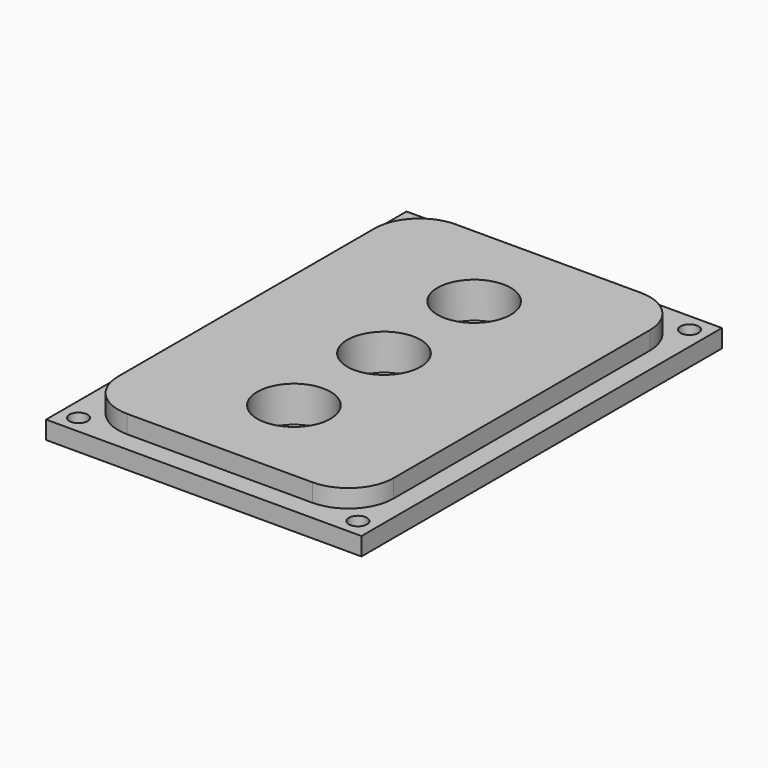
from build123d import *

# Parameters (mm, degrees)
F0_W            = 70
F0_H            = 100
F2_DEPTH        = 4
F1_W            = 61.1
F1_H            = 91.1
F3_DEPTH        = 4
F5_D            = 16.25
F5_DEPTH        = 10
F5_TIP          = 4.8819925296
F6_TEXT_SIZE    = 9.5338899996
F7_DEPTH        = 0.5
F9_R            = 10
F10_D           = 4
F10_DEPTH       = 10
F10_CSINK_D     = 5
F10_CSINK_ANGLE = 90
F10_TIP         = 1.2017212381


# Not quite as in the source:
# - Text() gives the source's letters only with a copy of the font that has no kerning and outlines rounded to 1/6400 em; it was checked with that copy


with BuildPart() as f2:
    # F0 (on Top) → F2 (new body)
    with BuildSketch(Plane.XY):
        Rectangle(F0_W, F0_H)
    extrude(amount=-F2_DEPTH)

    # F1 (on Top) → F3 (join)
    with BuildSketch(Plane.XY):
        Rectangle(F1_W, F1_H)
    extrude(amount=F3_DEPTH)

    # F5
    with Locations(Plane(origin=(0, 0, -4), x_dir=(1, 0, 0), z_dir=(0, 0, -1))):
        with Locations((0, 25), (0, 0), (0, -25)):
            Hole(F5_D / 2, depth=F5_DEPTH)
            with Locations((0, 0, -(F5_DEPTH + F5_TIP / 2))):  # 118° drill point
                Cone(0, F5_D / 2, F5_TIP, mode=Mode.SUBTRACT)

    # F6 (on face) → F7 (cut)
    with BuildSketch(Plane(origin=(0, 0, -4), x_dir=(1, 0, 0), z_dir=(0, 0, -1))):
        with Locations((-19, 40.1355992003)):
            Text('PRESS J8', F6_TEXT_SIZE, font='Open Sans', text_align=(TextAlign.LEFT, TextAlign.BOTTOM))
    extrude(amount=-F7_DEPTH, mode=Mode.SUBTRACT)

    # F9
    f9_edges = [f2.edges().sort_by_distance(p)[0] for p in [
        (-30.55, -45.55, 2),
        (30.55, -45.55, 2),
        (30.55, 45.55, 2),
        (-30.55, 45.55, 2),
    ]]
    fillet(f9_edges, radius=F9_R)

    # F10
    with Locations(Plane(origin=(0, 0, -4), x_dir=(1, 0, 0), z_dir=(0, 0, -1))):
        with Locations((-31, 46), (31, 46), (31, -46), (-31, -46)):
            CounterSinkHole(F10_D / 2, F10_CSINK_D / 2, depth=F10_DEPTH, counter_sink_angle=F10_CSINK_ANGLE)
            with Locations((0, 0, -(F10_DEPTH + F10_TIP / 2))):  # 118° drill point
                Cone(0, F10_D / 2, F10_TIP, mode=Mode.SUBTRACT)


solid = f2.part
